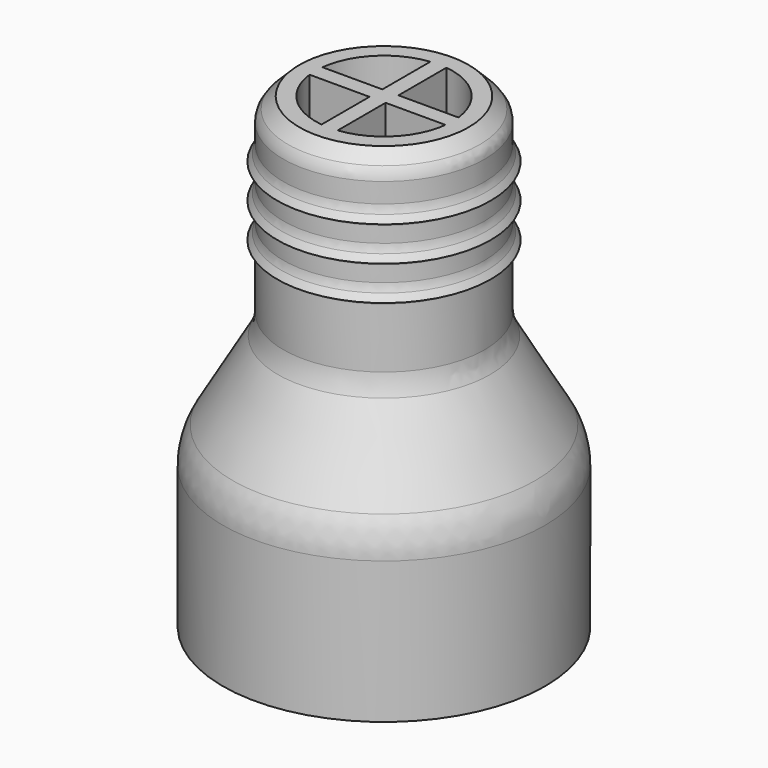
from build123d import *

# Parameters (mm, degrees)
F2_R      = 5
F3_R      = 9
F4_T      = -4
F7_SIZE   = 2
F8_R      = 2
F11_R     = 2
F12_R     = 0.5
F13_R     = 0.5
F14_W     = 2
F14_H     = 2
F15_DEPTH = 22
F16_R     = 0.9999


# Not quite as in the source:
# - a fillet or chamfer is up to 0.001 mm smaller than in the source, because OpenCascade refuses the exact size


with BuildPart() as f1:
    # F0 (on Front) → F1 (revolve)
    with BuildSketch(Plane.XZ):
        Polygon((0, 57.9903810568), (0, 0), (20, 0), (20, 20), (12.5, 32.9903810568), (12.5, 57.9903810568), align=None)
    revolve(axis=Axis((0, 0, 28.9951905284), (0, 0, 1)))

    # F2
    f2_edges = [f1.edges().sort_by_distance(p)[0] for p in [
        (-12.5, 0, 32.990381),
    ]]
    fillet(f2_edges, radius=F2_R)

    # F3
    f3_edges = [f1.edges().sort_by_distance(p)[0] for p in [
        (-20, 0, 20),
    ]]
    fillet(f3_edges, radius=F3_R)

    # F4
    f4_openings = [f1.faces().sort_by_distance(p)[0] for p in [
        (0, 0, 0),
        (0, 0, 57.990381),
    ]]
    offset(amount=F4_T, openings=f4_openings)

    # F5 (on Front) → F6 (revolve, cut)
    with BuildSketch(Plane.XZ):
        with BuildLine():
            ThreePointArc((16, 11.75), (16.8838834765, 12.1161165235), (17.25, 13))
            ThreePointArc((17.25, 13), (16.8838834765, 13.8838834765), (16, 14.25))
            Line((16, 14.25), (16, 11.75))
        make_face()
        with BuildLine():
            Line((16, 11.75), (16, 14.25))
            ThreePointArc((16, 14.25), (14.75, 13), (16, 11.75))
        make_face()
    revolve(axis=Axis((0, 0, 5.1447739825), (0, 0, 1)), mode=Mode.SUBTRACT)

    # F7
    f7_edges = [f1.edges().sort_by_distance(p)[0] for p in [
        (-16, 0, 0),
        (-12.5, 0, 57.990381),
    ]]
    chamfer(f7_edges, length=F7_SIZE)

    # F8
    f8_edges = [f1.edges().sort_by_distance(p)[0] for p in [
        (-16, 0, 2),
        (-12.5, 0, 55.990381),
    ]]
    fillet(f8_edges, radius=F8_R)

    # F9 (on Front) → F10 (revolve)
    with BuildSketch(Plane.XZ):
        Polygon((12.5, 52.161953932), (12.5, 50.8629158263), (13.25, 50.8629158263), align=None)
        Polygon((12.5, 47.8629158263), (12.5, 46.5638777207), (13.25, 46.5638777207), align=None)
        Polygon((12.5, 43.5638777207), (12.5, 42.264839615), (13.25, 42.264839615), align=None)
    revolve(axis=Axis((0, 0, 34.5272868872), (0, 0, 1)))

    # F11
    f11_edges = [f1.edges().sort_by_distance(p)[0] for p in [
        (-12.5, 0, 52.161954),
        (-12.5, 0, 47.862916),
        (-12.5, 0, 43.563878),
    ]]
    fillet(f11_edges, radius=F11_R)

    # F12
    f12_edges = [f1.edges().sort_by_distance(p)[0] for p in [
        (-12.5, 0, 50.862916),
        (-12.5, 0, 46.563878),
        (-12.5, 0, 42.26484),
    ]]
    fillet(f12_edges, radius=F12_R)

    # F13
    f13_edges = [f1.edges().sort_by_distance(p)[0] for p in [
        (-16, 0, 11.75),
    ]]
    fillet(f13_edges, radius=F13_R)

    # F14 (on face) → F15 (join)
    with BuildSketch(Plane.XY.offset(57.9903810568)):
        with BuildLine():
            ThreePointArc((-8.4409715081, 1), (-8.5, 0), (-8.4409715081, -1))
            Line((-8.4409715081, -1), (-1, -1))
            Line((-1, -1), (-1, 1))
            Line((-1, 1), (-8.4409715081, 1))
        make_face()
        Rectangle(F14_W, F14_H)
        with BuildLine():
            Line((-1, 8.4409715081), (-1, 1))
            Line((-1, 1), (1, 1))
            Line((1, 1), (1, 8.4409715081))
            ThreePointArc((1, 8.4409715081), (0, 8.5), (-1, 8.4409715081))
        make_face()
        with BuildLine():
            Line((1, 1), (1, -1))
            Line((1, -1), (8.4409715081, -1))
            ThreePointArc((8.4409715081, -1), (8.4852300446, -0.5008703332), (8.5, 0))
            ThreePointArc((8.5, 0), (8.4852300446, 0.5008703332), (8.4409715081, 1))
            Line((8.4409715081, 1), (1, 1))
        make_face()
        with BuildLine():
            Line((1, -1), (-1, -1))
            Line((-1, -1), (-1, -8.4409715081))
            ThreePointArc((-1, -8.4409715081), (0, -8.5), (1, -8.4409715081))
            Line((1, -8.4409715081), (1, -1))
        make_face()
    extrude(amount=-F15_DEPTH)

    # F16 (radius 1 in the source; OpenCascade refuses exactly that, so slightly less here)
    f16_edges = [f1.edges().sort_by_distance(p)[0] for p in [
        (1, 4.720486, 35.990381),
        (-1, 4.720486, 35.990381),
        (4.720486, 1, 35.990381),
        (4.720486, -1, 35.990381),
        (1, -4.720486, 35.990381),
        (-1, -4.720486, 35.990381),
        (-4.720486, -1, 35.990381),
        (-4.720486, 1, 35.990381),
    ]]
    fillet(f16_edges, radius=F16_R)


solid = f1.part
